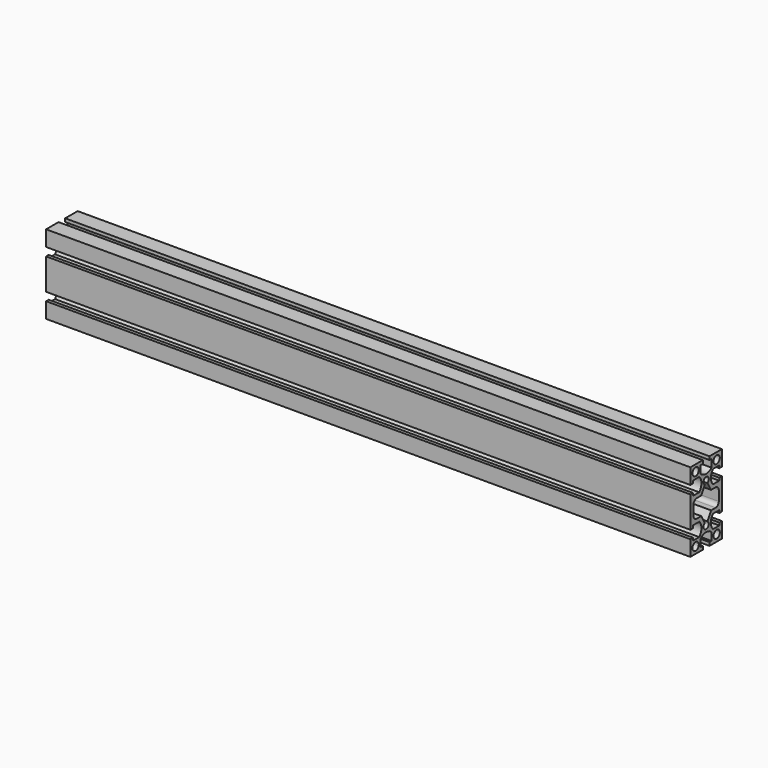
from build123d import *

# Parameters (mm, degrees)
F0_R     = 3
F1_DEPTH = 490


# Not quite as in the source:
# - ends of sketch curves that miss each other by under 0.0002 mm in the source are joined


with BuildPart() as f1:
    # F0 (on Right) → F1 (new body)
    with BuildSketch(Plane.YZ):
        with BuildLine():
            Line((12.5, -11.85), (15, -11.85))
            Line((15, -11.85), (15, 11.85))
            Line((15, 11.85), (12.5, 11.85))
            Line((12.5, 11.85), (12.5, 9.85))
            Line((12.5, 9.85), (6.547707, 9.85))
            ThreePointArc((6.5477069495, 9.8499999523), (4.5, 15), (6.5477069495, 20.1500000477))
            Line((6.547707, 20.15), (12.5, 20.15))
            Line((12.5, 20.15), (12.5, 18.15))
            Line((12.5, 18.15), (15, 18.15))
            Line((15, 18.15), (15, 30))
            Line((15, 30), (3.15, 30))
            Line((3.15, 30), (3.15, 27.5))
            Line((3.15, 27.5), (5.15, 27.5))
            Line((5.15, 27.5), (5.15, 21.547707))
            ThreePointArc((5.1500000477, 21.5477069495), (0, 19.5), (-5.1500000477, 21.5477069495))
            Line((-5.15, 21.547707), (-5.15, 27.5))
            Line((-5.15, 27.5), (-3.15, 27.5))
            Line((-3.15, 27.5), (-3.15, 30))
            Line((-3.15, 30), (-15, 30))
            Line((-15, 30), (-15, 18.15))
            Line((-15, 18.15), (-12.5, 18.15))
            Line((-12.5, 18.15), (-12.5, 20.15))
            Line((-12.5, 20.15), (-6.547707, 20.15))
            ThreePointArc((-6.5477069495, 20.1500000477), (-4.5, 15), (-6.5477069495, 9.8499999523))
            Line((-6.547707, 9.85), (-12.5, 9.85))
            Line((-12.5, 9.85), (-12.5, 11.85))
            Line((-12.5, 11.85), (-15, 11.85))
            Line((-15, 11.85), (-15, -11.85))
            Line((-15, -11.85), (-12.5, -11.85))
            Line((-12.5, -11.85), (-12.5, -9.85))
            Line((-12.5, -9.85), (-6.547707, -9.85))
            ThreePointArc((-6.5477069495, -9.8499999523), (-4.5, -15), (-6.5477069495, -20.1500000477))
            Line((-6.547707, -20.15), (-12.5, -20.15))
            Line((-12.5, -20.15), (-12.5, -18.15))
            Line((-12.5, -18.15), (-15, -18.15))
            Line((-15, -18.15), (-15, -30))
            Line((-15, -30), (-3.15, -30))
            Line((-3.15, -30), (-3.15, -27.5))
            Line((-3.15, -27.5), (-5.15, -27.5))
            Line((-5.15, -27.5), (-5.15, -21.547707))
            ThreePointArc((-5.1500000477, -21.5477069495), (0, -19.5), (5.1500000477, -21.5477069495))
            Line((5.15, -21.547707), (5.15, -27.5))
            Line((5.15, -27.5), (3.15, -27.5))
            Line((3.15, -27.5), (3.15, -30))
            Line((3.15, -30), (15, -30))
            Line((15, -30), (15, -18.15))
            Line((15, -18.15), (12.5, -18.15))
            Line((12.5, -18.15), (12.5, -20.15))
            Line((12.5, -20.15), (6.547707, -20.15))
            ThreePointArc((6.5477069495, -20.1500000477), (4.5, -15), (6.5477069495, -9.8499999523))
            Line((6.547707, -9.85), (12.5, -9.85))
            Line((12.5, -9.85), (12.5, -11.85))
        make_face()
        with Locations((-10, -25)):
            Circle(F0_R, mode=Mode.SUBTRACT)
        with Locations((10, -25)):
            Circle(F0_R, mode=Mode.SUBTRACT)
        with Locations((-10, 25)):
            Circle(F0_R, mode=Mode.SUBTRACT)
        with BuildLine():
            ThreePointArc((-12, 3.85), (-11.1213203436, 5.9713203436), (-9, 6.85))
            Line((-9, 6.85), (-4.705405, 6.85))
            Line((-4.705405, 6.85), (-1.25, 12.834936))
            ThreePointArc((-1.25, 12.834936), (0, 17.5), (1.2499997876, 12.8349363679))
            Line((1.2499997876, 12.8349363679), (4.705405, 6.85))
            Line((4.705405, 6.85), (9, 6.85))
            ThreePointArc((9, 6.85), (11.1213203436, 5.9713203436), (12, 3.85))
            Line((12, 3.85), (12, -3.85))
            ThreePointArc((12, -3.85), (11.1213203436, -5.9713203436), (9, -6.85))
            Line((9, -6.85), (4.705405, -6.85))
            Line((4.705405, -6.85), (1.25, -12.834937))
            ThreePointArc((1.25, -12.834937), (0, -17.5), (-1.2500002206, -12.8349366179))
            Line((-1.2500002206, -12.8349366179), (-4.705405, -6.85))
            Line((-4.705405, -6.85), (-9, -6.85))
            ThreePointArc((-9, -6.85), (-11.1213203436, -5.9713203436), (-12, -3.85))
            Line((-12, -3.85), (-12, 3.85))
        make_face(mode=Mode.SUBTRACT)
        with Locations((10, 25)):
            Circle(F0_R, mode=Mode.SUBTRACT)
    extrude(amount=F1_DEPTH)


solid = f1.part
